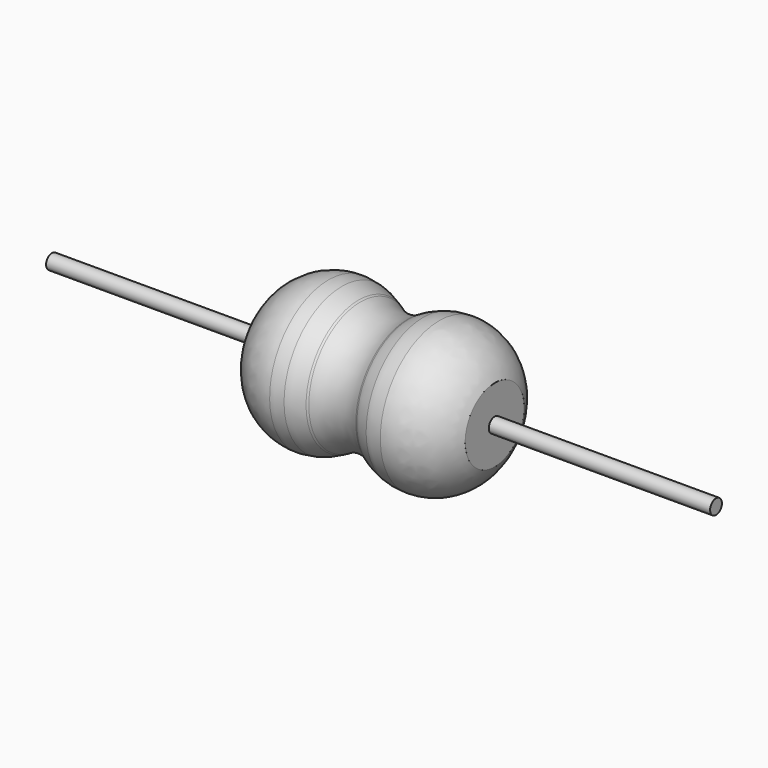
from build123d import *

# Parameters (mm, degrees)
F0_W = 30
F0_H = 1


# Not quite as in the source:
# - a feature names something its author has since deleted; it is built from what else it names
# - the program builds the solid bodies; features that only make, move or delete a surface that nothing else refers to are left out


with BuildPart() as f1:
    # F0 (on Front) → F1 (revolve)
    with BuildSketch(Plane.XZ):
        Polygon((0, 1), (0, 0), (30, 0), (30, 1), (30, 5), (0, 5), align=None)
        with BuildLine():
            ThreePointArc((7.5, 10), (2.9930609057, 8.6354086415), (0, 5))
            Line((0, 5), (30, 5))
            ThreePointArc((30, 5), (27.0069390843, 8.6354086482), (22.4999999759, 10))
            ThreePointArc((22.4999999759, 10), (21.4125129517, 9.9268939958), (20.3445956085, 9.7088915559))
            ThreePointArc((20.3445956085, 9.7088915559), (19.3760252959, 9.3754271244), (18.457110969, 8.9227424246))
            ThreePointArc((18.457110969, 8.9227424246), (18.3206839191, 8.8427070903), (18.185840708, 8.7600311984))
            ThreePointArc((18.185840708, 8.7600311984), (15, 7.8443619295), (11.814159292, 8.7600311984))
            ThreePointArc((11.814159292, 8.7600311984), (11.6898538017, 8.8363755911), (11.5641977003, 8.9104759649))
            ThreePointArc((11.5641977003, 8.9104759649), (10.4634096842, 9.4403042268), (9.2956262041, 9.7990994148))
            ThreePointArc((9.2956262041, 9.7990994148), (8.4034149808, 9.9496186518), (7.5, 10))
        make_face()
    revolve(axis=Axis((15, 0, 0), (1, 0, 0)))


with BuildPart() as f2:
    # F0 (on Front) → F2 (revolve)
    with BuildSketch(Plane.XZ):
        with Locations((-15, 0.5)):
            Rectangle(F0_W, F0_H)
    revolve(axis=Axis((15, 0, 0), (1, 0, 0)))


with BuildPart() as f2b:
    # F0 (on Front) → F2, piece 2 (revolve)
    with BuildSketch(Plane.XZ):
        with Locations((45, 0.5)):
            Rectangle(F0_W, F0_H)
    revolve(axis=Axis((15, 0, 0), (1, 0, 0)))


solid = Compound([f1.part, f2.part, f2b.part])
